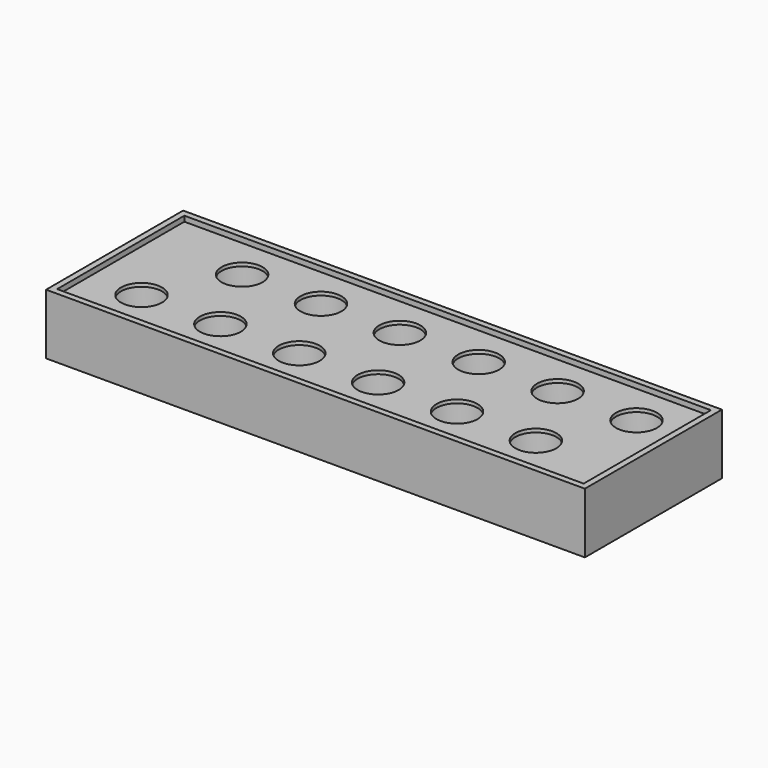
from build123d import *

# Parameters (mm, degrees)
F0_W     = 156.1555638909
F0_H     = 49.64682227
F0_W_2   = 152.5995656848
F0_H_2   = 46.0908240639
F1_DEPTH = 2.54
F0_R     = 10.5160009116
F0_R_2   = 9.5
F2_DEPTH = 10
F0_R_3   = 5.944
F0_R_4   = 5.9439986944
F3_DEPTH = 1
F4_DEPTH = 15


with BuildPart() as f1:
    # F0 (on Top) → F1 (new body)
    with BuildSketch(Plane.XY):
        with Locations((3.8024671376, 31.7355815787)):
            Rectangle(F0_W, F0_H)
        with Locations((3.8024671376, 31.7355815787)):
            Rectangle(F0_W_2, F0_H_2, mode=Mode.SUBTRACT)
    extrude(amount=F1_DEPTH)

    # F0 (on Top) → F4 (join)
    with BuildSketch(Plane.XY):
        with Locations((3.8024671376, 31.7355815787)):
            Rectangle(F0_W, F0_H)
        with Locations((3.8024671376, 31.7355815787)):
            Rectangle(F0_W_2, F0_H_2, mode=Mode.SUBTRACT)
    extrude(amount=-F4_DEPTH)


with BuildPart() as f2:
    # F0 (on Top) → F2 (new body)
    with BuildSketch(Plane.XY):
        with Locations((-46.0894259106, 42.6910893638)):
            Circle(F0_R)
        with Locations((-46.0894259106, 42.6910893638)):
            Circle(F0_R_2, mode=Mode.SUBTRACT)
    extrude(amount=-F2_DEPTH)


with BuildPart() as f2b:
    # F0 (on Top) → F2, piece 2 (new body)
    with BuildSketch(Plane.XY):
        with Locations((-57.6259419322, 20.666833967)):
            Circle(F0_R)
        with Locations((-57.6259419322, 20.666833967)):
            Circle(F0_R_2, mode=Mode.SUBTRACT)
    extrude(amount=-F2_DEPTH)


with BuildPart() as f2c:
    # F0 (on Top) → F2, piece 3 (new body)
    with BuildSketch(Plane.XY):
        with Locations((-34.7659419322, 20.666833967)):
            Circle(F0_R)
        with Locations((-34.7659419322, 20.666833967)):
            Circle(F0_R_2, mode=Mode.SUBTRACT)
    extrude(amount=-F2_DEPTH)


with BuildPart() as f2d:
    # F0 (on Top) → F2, piece 4 (new body)
    with BuildSketch(Plane.XY):
        with Locations((-23.2294259106, 42.6910893638)):
            Circle(F0_R)
        with Locations((-23.2294259106, 42.6910893638)):
            Circle(F0_R_2, mode=Mode.SUBTRACT)
    extrude(amount=-F2_DEPTH)


with BuildPart() as f2e:
    # F0 (on Top) → F2, piece 5 (new body)
    with BuildSketch(Plane.XY):
        with Locations((-0.3694259106, 42.6910893638)):
            Circle(F0_R)
        with Locations((-0.3694259106, 42.6910893638)):
            Circle(F0_R_2, mode=Mode.SUBTRACT)
    extrude(amount=-F2_DEPTH)


with BuildPart() as f2f:
    # F0 (on Top) → F2, piece 6 (new body)
    with BuildSketch(Plane.XY):
        with Locations((-11.9059419322, 20.666833967)):
            Circle(F0_R)
        with Locations((-11.9059419322, 20.666833967)):
            Circle(F0_R_2, mode=Mode.SUBTRACT)
    extrude(amount=-F2_DEPTH)


with BuildPart() as f2g:
    # F0 (on Top) → F2, piece 7 (new body)
    with BuildSketch(Plane.XY):
        with Locations((10.9540580678, 20.666833967)):
            Circle(F0_R)
        with Locations((10.9540580678, 20.666833967)):
            Circle(F0_R_2, mode=Mode.SUBTRACT)
    extrude(amount=-F2_DEPTH)


with BuildPart() as f2h:
    # F0 (on Top) → F2, piece 8 (new body)
    with BuildSketch(Plane.XY):
        with Locations((22.4905740894, 42.6910893638)):
            Circle(F0_R)
        with Locations((22.4905740894, 42.6910893638)):
            Circle(F0_R_2, mode=Mode.SUBTRACT)
    extrude(amount=-F2_DEPTH)


with BuildPart() as f2i:
    # F0 (on Top) → F2, piece 9 (new body)
    with BuildSketch(Plane.XY):
        with Locations((33.8140580678, 20.666833967)):
            Circle(F0_R)
        with Locations((33.8140580678, 20.666833967)):
            Circle(F0_R_2, mode=Mode.SUBTRACT)
    extrude(amount=-F2_DEPTH)


with BuildPart() as f2j:
    # F0 (on Top) → F2, piece 10 (new body)
    with BuildSketch(Plane.XY):
        with Locations((45.3505740894, 42.6910893638)):
            Circle(F0_R)
        with Locations((45.3505740894, 42.6910893638)):
            Circle(F0_R_2, mode=Mode.SUBTRACT)
    extrude(amount=-F2_DEPTH)


with BuildPart() as f2k:
    # F0 (on Top) → F2, piece 11 (new body)
    with BuildSketch(Plane.XY):
        with Locations((56.6740580678, 20.666833967)):
            Circle(F0_R)
        with Locations((56.6740580678, 20.666833967)):
            Circle(F0_R_2, mode=Mode.SUBTRACT)
    extrude(amount=-F2_DEPTH)


with BuildPart() as f2l:
    # F0 (on Top) → F2, piece 12 (new body)
    with BuildSketch(Plane.XY):
        with Locations((68.2105740894, 42.6910893638)):
            Circle(F0_R)
        with Locations((68.2105740894, 42.6910893638)):
            Circle(F0_R_2, mode=Mode.SUBTRACT)
    extrude(amount=-F2_DEPTH)


with BuildPart() as f3:
    # F0 (on Top) → F3 (new body)
    with BuildSketch(Plane.XY):
        with Locations((3.8024671376, 31.7355815787)):
            Rectangle(F0_W_2, F0_H_2)
        with Locations((-57.6259419322, 20.666833967)):
            Circle(F0_R, mode=Mode.SUBTRACT)
        with Locations((-34.7659419322, 20.666833967)):
            Circle(F0_R, mode=Mode.SUBTRACT)
        with Locations((-11.9059419322, 20.666833967)):
            Circle(F0_R, mode=Mode.SUBTRACT)
        with Locations((10.9540580678, 20.666833967)):
            Circle(F0_R, mode=Mode.SUBTRACT)
        with Locations((33.8140580678, 20.666833967)):
            Circle(F0_R, mode=Mode.SUBTRACT)
        with Locations((56.6740580678, 20.666833967)):
            Circle(F0_R, mode=Mode.SUBTRACT)
        with Locations((-46.0894259106, 42.6910893638)):
            Circle(F0_R, mode=Mode.SUBTRACT)
        with Locations((-23.2294259106, 42.6910893638)):
            Circle(F0_R, mode=Mode.SUBTRACT)
        with Locations((-0.3694259106, 42.6910893638)):
            Circle(F0_R, mode=Mode.SUBTRACT)
        with Locations((22.4905740894, 42.6910893638)):
            Circle(F0_R, mode=Mode.SUBTRACT)
        with Locations((45.3505740894, 42.6910893638)):
            Circle(F0_R, mode=Mode.SUBTRACT)
        with Locations((68.2105740894, 42.6910893638)):
            Circle(F0_R, mode=Mode.SUBTRACT)
        with Locations((-46.0894259106, 42.6910893638)):
            Circle(F0_R)
        with Locations((-46.0894259106, 42.6910893638)):
            Circle(F0_R_2, mode=Mode.SUBTRACT)
        with Locations((-57.6259419322, 20.666833967)):
            Circle(F0_R)
        with Locations((-57.6259419322, 20.666833967)):
            Circle(F0_R_2, mode=Mode.SUBTRACT)
        with Locations((-34.7659419322, 20.666833967)):
            Circle(F0_R)
        with Locations((-34.7659419322, 20.666833967)):
            Circle(F0_R_2, mode=Mode.SUBTRACT)
        with Locations((-23.2294259106, 42.6910893638)):
            Circle(F0_R)
        with Locations((-23.2294259106, 42.6910893638)):
            Circle(F0_R_2, mode=Mode.SUBTRACT)
        with Locations((-0.3694259106, 42.6910893638)):
            Circle(F0_R)
        with Locations((-0.3694259106, 42.6910893638)):
            Circle(F0_R_2, mode=Mode.SUBTRACT)
        with Locations((10.9540580678, 20.666833967)):
            Circle(F0_R)
        with Locations((10.9540580678, 20.666833967)):
            Circle(F0_R_2, mode=Mode.SUBTRACT)
        with Locations((-11.9059419322, 20.666833967)):
            Circle(F0_R)
        with Locations((-11.9059419322, 20.666833967)):
            Circle(F0_R_2, mode=Mode.SUBTRACT)
        with Locations((56.6740580678, 20.666833967)):
            Circle(F0_R)
        with Locations((56.6740580678, 20.666833967)):
            Circle(F0_R_2, mode=Mode.SUBTRACT)
        with Locations((45.3505740894, 42.6910893638)):
            Circle(F0_R)
        with Locations((45.3505740894, 42.6910893638)):
            Circle(F0_R_2, mode=Mode.SUBTRACT)
        with Locations((22.4905740894, 42.6910893638)):
            Circle(F0_R)
        with Locations((22.4905740894, 42.6910893638)):
            Circle(F0_R_2, mode=Mode.SUBTRACT)
        with Locations((33.8140580678, 20.666833967)):
            Circle(F0_R)
        with Locations((33.8140580678, 20.666833967)):
            Circle(F0_R_2, mode=Mode.SUBTRACT)
        with Locations((68.2105740894, 42.6910893638)):
            Circle(F0_R)
        with Locations((68.2105740894, 42.6910893638)):
            Circle(F0_R_2, mode=Mode.SUBTRACT)
        with Locations((-46.0894259106, 42.6910893638)):
            Circle(F0_R_2)
        with Locations((-46.0894259106, 42.6910893638)):
            Circle(F0_R_3, mode=Mode.SUBTRACT)
        with Locations((-23.2294259106, 42.6910893638)):
            Circle(F0_R_2)
        with Locations((-23.2294259106, 42.6910893638)):
            Circle(F0_R_3, mode=Mode.SUBTRACT)
        with Locations((-57.6259419322, 20.666833967)):
            Circle(F0_R_2)
        with Locations((-57.6259419322, 20.666833967)):
            Circle(F0_R_4, mode=Mode.SUBTRACT)
        with Locations((-34.7659419322, 20.666833967)):
            Circle(F0_R_2)
        with Locations((-34.7659419322, 20.666833967)):
            Circle(F0_R_3, mode=Mode.SUBTRACT)
        with Locations((-11.9059419322, 20.666833967)):
            Circle(F0_R_2)
        with Locations((-11.9059419322, 20.666833967)):
            Circle(F0_R_3, mode=Mode.SUBTRACT)
        with Locations((-0.3694259106, 42.6910893638)):
            Circle(F0_R_2)
        with Locations((-0.3694259106, 42.6910893638)):
            Circle(F0_R_3, mode=Mode.SUBTRACT)
        with Locations((22.4905740894, 42.6910893638)):
            Circle(F0_R_2)
        with Locations((22.4905740894, 42.6910893638)):
            Circle(F0_R_3, mode=Mode.SUBTRACT)
        with Locations((10.9540580678, 20.666833967)):
            Circle(F0_R_2)
        with Locations((10.9540580678, 20.666833967)):
            Circle(F0_R_3, mode=Mode.SUBTRACT)
        with Locations((33.8140580678, 20.666833967)):
            Circle(F0_R_2)
        with Locations((33.8140580678, 20.666833967)):
            Circle(F0_R_3, mode=Mode.SUBTRACT)
        with Locations((45.3505740894, 42.6910893638)):
            Circle(F0_R_2)
        with Locations((45.3505740894, 42.6910893638)):
            Circle(F0_R_3, mode=Mode.SUBTRACT)
        with Locations((56.6740580678, 20.666833967)):
            Circle(F0_R_2)
        with Locations((56.6740580678, 20.666833967)):
            Circle(F0_R_3, mode=Mode.SUBTRACT)
        with Locations((68.2105740894, 42.6910893638)):
            Circle(F0_R_2)
        with Locations((68.2105740894, 42.6910893638)):
            Circle(F0_R_3, mode=Mode.SUBTRACT)
    extrude(amount=F3_DEPTH)


solid = Compound([f1.part, f2.part, f2b.part, f2c.part, f2d.part, f2e.part, f2f.part, f2g.part, f2h.part, f2i.part, f2j.part, f2k.part, f2l.part, f3.part])
